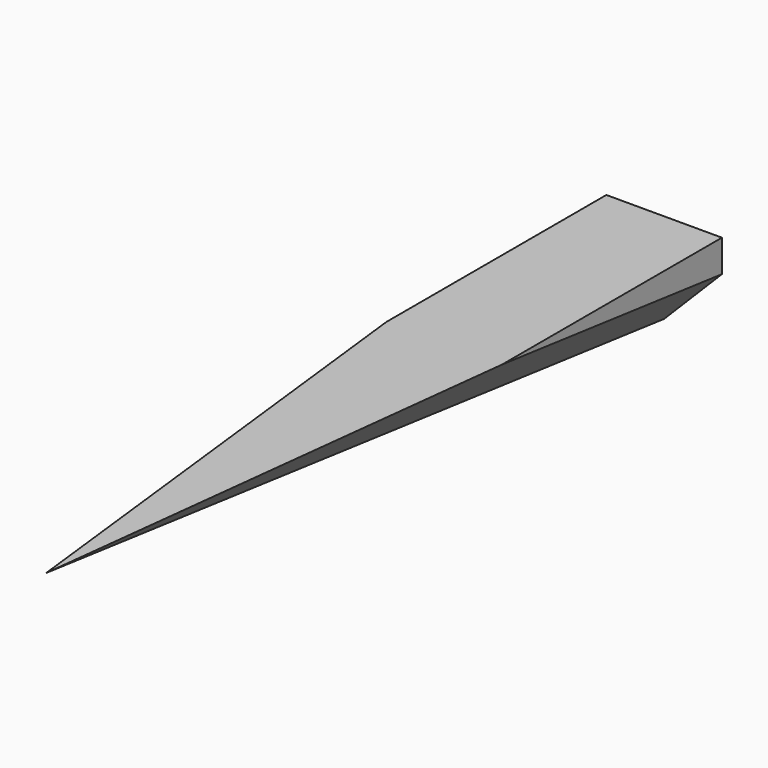
from build123d import *

# Parameters (mm, degrees)
F1_DEPTH = 10.16
F2_SIZE  = 5.07999


# Not quite as in the source:
# - a fillet or chamfer is up to 0.001 mm smaller than in the source, because OpenCascade refuses the exact size


with BuildPart() as f1:
    # F0 (on Right) → F1 (new body)
    with BuildSketch(Plane.YZ):
        Polygon((-45.6850975752, 0), (22.2317874432, -7.939924486), (22.2317874432, 0), align=None)
    extrude(amount=F1_DEPTH)

    # F2 (size 5.08 in the source; OpenCascade refuses exactly that, so slightly less here)
    f2_edges = [f1.edges().sort_by_distance(p)[0] for p in [
        (10.16, -11.726655, -3.969962),
        (0, -11.726655, -3.969962),
    ]]
    chamfer(f2_edges, length=F2_SIZE)


solid = f1.part
